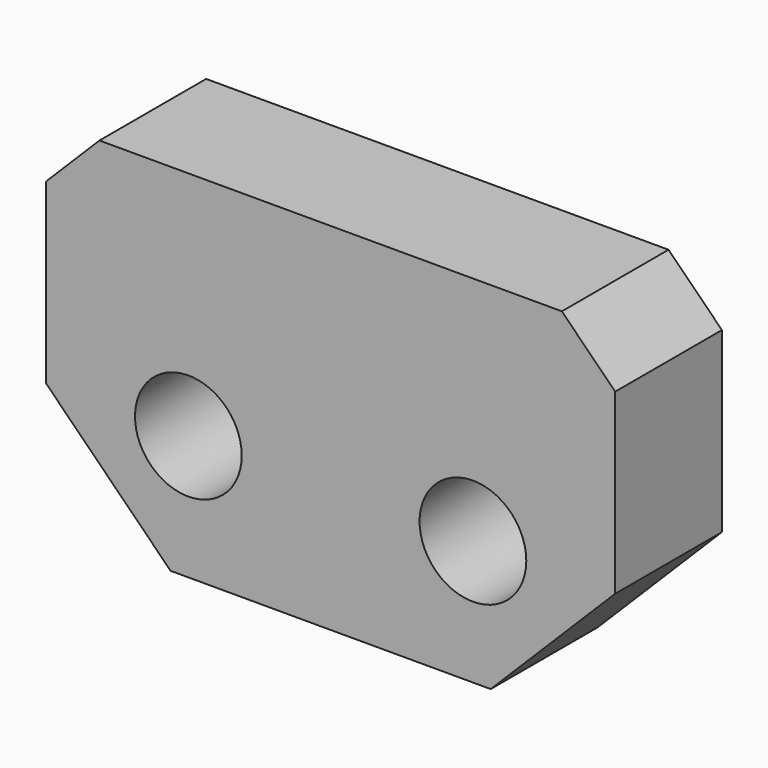
from build123d import *

# Parameters (mm, degrees)
F1_W     = 32
F1_H     = 20
F2_DEPTH = 7.5
F3_SIZE  = 7
F4_R     = 3
F5_DEPTH = 25
F6_SIZE  = 3
F7_W     = 10
F7_H     = 2
F8_DEPTH = 5
F9_SIZE2 = 0.99999
F9_SIZE  = 4.99999


# Not quite as in the source:
# - a fillet or chamfer is up to 0.001 mm smaller than in the source, because OpenCascade refuses the exact size


with BuildPart() as f2:
    # F1 (on Front) → F2 (new body)
    with BuildSketch(Plane.XZ):
        Rectangle(F1_W, F1_H)
    extrude(amount=F2_DEPTH)

    # F3
    f3_edges = [f2.edges().sort_by_distance(p)[0] for p in [
        (-16, -3.75, -10),
        (16, -3.75, -10),
    ]]
    chamfer(f3_edges, length=F3_SIZE)

    # F4 (on face) → F5 (cut)
    with BuildSketch(Plane.XZ.offset(7.5)):
        with Locations((-8, -3)):
            Circle(F4_R)
        with Locations((8, -3)):
            Circle(F4_R)
    extrude(amount=-F5_DEPTH, mode=Mode.SUBTRACT)

    # F6
    f6_edges = [f2.edges().sort_by_distance(p)[0] for p in [
        (16, -3.75, 10),
        (-16, -3.75, 10),
    ]]
    chamfer(f6_edges, length=F6_SIZE)

    # F7 (on face) → F8 (cut)
    with BuildSketch(Plane(origin=(0, 0, -10), x_dir=(1, 0, 0), z_dir=(0, 0, -1))):
        with Locations((0, 4.75)):
            Rectangle(F7_W, F7_H)
        with Locations((0, 2.75)):
            Rectangle(F7_W, F7_H)
    extrude(amount=-F8_DEPTH, mode=Mode.SUBTRACT)

    # F9 (size 5 and 1 in the source; OpenCascade refuses exactly that, so slightly less here)
    f9_edges = [f2.edges().sort_by_distance(p)[0] for p in [
        (0, -1.75, -5),
        (0, -5.75, -5),
    ]]
    chamfer(f9_edges, length=F9_SIZE, length2=F9_SIZE2)


solid = f2.part
